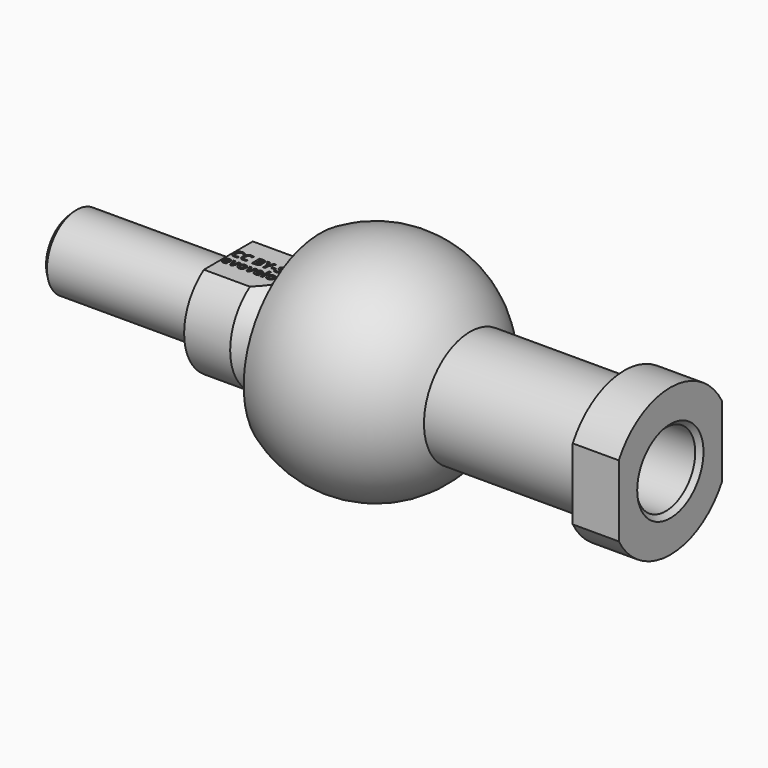
from build123d import *

# Parameters (mm, degrees)
F4_DEPTH      = 5
F5_D          = 8
F5_DEPTH      = 16
F5_TIP        = 2.4034424761
F6_D          = 6.5
F6_DEPTH      = 4
F6_START      = 16.4506455
F6_TIP        = 1.9527970118
F7_D          = 2
F9_DEPTH      = 6.8390457188
F10_SIZE      = 0.5
F10_2_SIZE    = 0.5
F11_TEXT_SIZE = 1.4945277879
F12_DEPTH     = 0.2


# Not quite as in the source:
# - Text() gives the source's letters only with a copy of the font that has no kerning and outlines rounded to 1/6400 em; it was checked with that copy


with BuildPart() as f1:
    # F0 (on Top) → F1 (revolve)
    with BuildSketch(Plane.XY):
        with BuildLine():
            ThreePointArc((-6.0445384271, 5.7607339118), (3.1024670936, 7.7522382531), (8.35, 0))
            Line((8.35, 0), (32, 0))
            Line((32, 0), (32, 8))
            Line((32, 8), (27, 8))
            Line((27, 8), (27, 6.25))
            Line((27, 6.25), (10.2439006243, 6.25))
            ThreePointArc((10.2439006243, 6.25), (2.9402342816, 11.6342177378), (-6.0445384271, 10.3664630035))
            Line((-6.0445384271, 10.3664630035), (-6.0445384271, 5.7607339118))
        make_face()
    revolve(axis=Axis((5.2878996746, 0, 0), (1, 0, 0)))

    # F3 (on face) → F4 (cut, through all)
    with BuildSketch(Plane.YZ.offset(32)):
        with BuildLine():
            ThreePointArc((8, 0), (7.7459666924, 2), (7, 3.8729833462))
            Line((7, 3.8729833462), (7, -3.8729833462))
            ThreePointArc((7, -3.8729833462), (7.7459666924, -2), (8, 0))
        make_face()
        with BuildLine():
            Line((-7, -3.8729833462), (-7, 3.8729833462))
            ThreePointArc((-7, 3.8729833462), (-8, 0), (-7, -3.8729833462))
        make_face()
    extrude(amount=-F4_DEPTH, mode=Mode.SUBTRACT)

    # F5
    with Locations(Plane.YZ.offset(32)):
        with Locations((0, 0)):
            Hole(F5_D / 2, depth=F5_DEPTH)
            with Locations((0, 0, -(F5_DEPTH + F5_TIP / 2))):  # 118° drill point
                Cone(0, F5_D / 2, F5_TIP, mode=Mode.SUBTRACT)

    # F6
    # its depths count from where the whole tool has entered the part; down to there all is cleared
    with Locations(Plane.YZ.offset(32)):
        with Locations((0, 0)):
            Hole(F6_D / 2, depth=F6_START)
    with Locations(Plane.YZ.offset(32).offset(-F6_START)):
        with Locations((0, 0)):
            Hole(F6_D / 2, depth=F6_DEPTH)
            with Locations((0, 0, -(F6_DEPTH + F6_TIP / 2))):  # 118° drill point
                Cone(0, F6_D / 2, F6_TIP, mode=Mode.SUBTRACT)

    # F7 (through all)
    with Locations(Plane.YZ.offset(32)):
        with Locations((0, 0)):
            Hole(F7_D / 2)

    # F10#2
    f10_2_edges = [f1.edges().sort_by_distance(p)[0] for p in [
        (32, -4, 0),
    ]]
    chamfer(f10_2_edges, length=F10_2_SIZE)


with BuildPart() as f2:
    # F0 (on Top) → F2 (revolve)
    with BuildSketch(Plane.XY):
        with BuildLine():
            Line((-33, 0), (8.35, 0))
            ThreePointArc((8.35, 0), (3.1024670936, 7.7522382531), (-6.0445384271, 5.7607339118))
            ThreePointArc((-6.0445384271, 5.7607339118), (-6.7447532249, 4.92247945), (-7.3295634249, 4))
            Line((-7.3295634249, 4), (-11, 6.003086057))
            Line((-11, 6.003086057), (-16, 6.003086057))
            Line((-16, 6.003086057), (-16, 4))
            Line((-16, 4), (-33, 4))
            Line((-33, 4), (-33, 0))
        make_face()
    revolve(axis=Axis((5.2878996746, 0, 0), (1, 0, 0)))

    # F8 (on face) → F9 (cut, through all)
    with BuildSketch(Plane(origin=(-16, 0, 0), x_dir=(0, -1, 0), z_dir=(-1, 0, 0))):
        with BuildLine():
            ThreePointArc((3.3222044199, 5), (0, 6.003086057), (-3.3222044199, 5))
            Line((-3.3222044199, 5), (3.3222044199, 5))
        make_face()
        with BuildLine():
            Line((3.3222044199, -5), (-3.3222044199, -5))
            ThreePointArc((-3.3222044199, -5), (0, -6.003086057), (3.3222044199, -5))
        make_face()
    extrude(amount=-F9_DEPTH, mode=Mode.SUBTRACT)

    # F10
    f10_edges = [f2.edges().sort_by_distance(p)[0] for p in [
        (-33, -4, 0),
    ]]
    chamfer(f10_edges, length=F10_SIZE)

    # F11 (on face) → F12 (cut)
    with BuildSketch(Plane.XY.offset(5)):
        with Locations((-16, 0.1542052578)):
            Text('CC BY-SA', F11_TEXT_SIZE, font='Open Sans', font_style=FontStyle.BOLD, text_align=(TextAlign.LEFT, TextAlign.BOTTOM))
        with Locations((-16, -1.2673561234)):
            Text('evovelo', F11_TEXT_SIZE, font='Open Sans', font_style=FontStyle.BOLD, text_align=(TextAlign.LEFT, TextAlign.BOTTOM))
    extrude(amount=-F12_DEPTH, mode=Mode.SUBTRACT)


solid = Compound([f1.part, f2.part])
